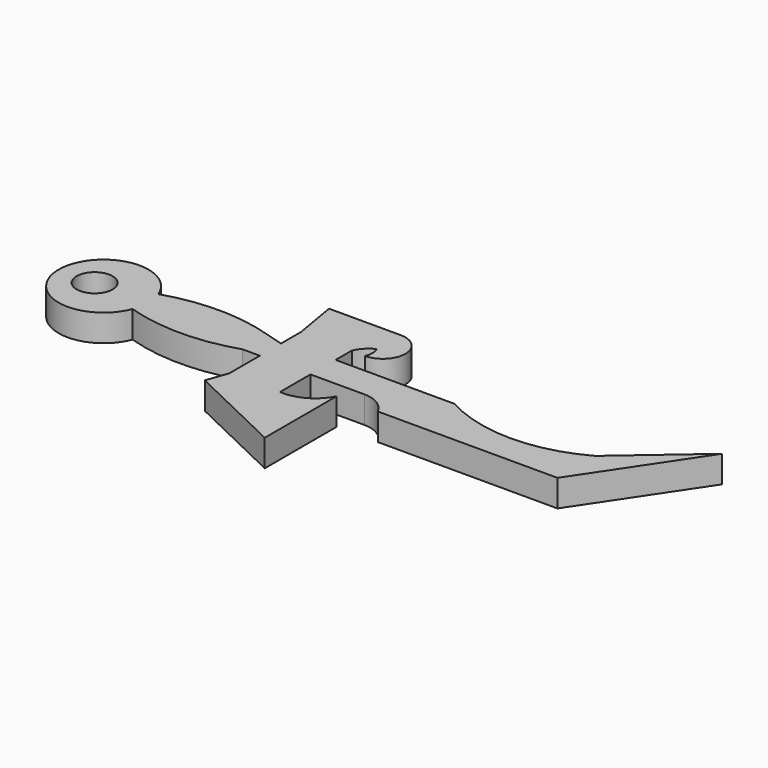
from build123d import *

# Parameters (mm, degrees)
F1_DEPTH = 3
F3_D     = 4


# Not quite as in the source:
# - a feature names something its author has since deleted; it is built from what else it names


with BuildPart() as f1:
    # F0 (on Top) → F1 (new body)
    with BuildSketch(Plane.XY):
        with BuildLine():
            Line((14.0881506171, 0), (14.0881506171, 3.5))
            ThreePointArc((14.0881506171, 3.5), (7.9876115371, 4.4807007673), (1.8788639221, 3.5525016304))
            ThreePointArc((1.8788639221, 3.5525016304), (2.1302987541, 2.666794093), (2.2150684857, 1.75))
            ThreePointArc((2.2150684857, 1.75), (2.1302987541, 0.833205907), (1.8788639221, -0.0525016304))
            ThreePointArc((1.8788639221, -0.0525016304), (7.9876115371, -0.9807007673), (14.0881506171, 0))
        make_face()
        with BuildLine():
            Line((21.6484292713, 3.5), (21.6484292713, 0))
            Line((21.6484292713, 0), (27.6484292713, 0))
            ThreePointArc((27.6484292713, 0), (29.3682210792, -0.4835632197), (30.5839958787, -1.7925356741))
            Line((30.5839958787, -1.7925356741), (50.5839958787, -1.7925356741))
            Line((50.5839958787, -1.7925356741), (58.9184745012, 10.6788903105))
            Line((58.9184745012, 10.6788903105), (50.5839958787, 3.5))
            ThreePointArc((50.5839958787, 3.5), (42.7439688076, 1.4762635236), (34.9039417364, 3.5))
            Line((34.9039417364, 3.5), (21.6484292713, 3.5))
        make_face()
        with BuildLine():
            Line((16.0120092332, 2.9430498835), (14.0881506171, 3.5))
            Line((14.0881506171, 3.5), (14.0881506171, 0))
            Line((14.0881506171, 0), (16.0120092332, 0))
            Line((16.0120092332, 0), (16.0120092332, -4.25))
            Line((16.0120092332, -4.25), (15.1717471866, -6.6045614651))
            Line((15.1717471866, -6.6045614651), (25.9923258961, -11.7925356741))
            Line((25.9923258961, -11.7925356741), (25.9923258961, -1.7925356741))
            ThreePointArc((25.9923258961, -1.7925356741), (24.192277602, -3.6786508222), (21.6484292713, -4.25))
            Line((21.6484292713, -4.25), (21.6484292713, 0))
            Line((21.6484292713, 0), (21.6484292713, 3.5))
            Line((21.6484292713, 3.5), (21.6484292713, 5.75))
            ThreePointArc((21.6484292713, 5.75), (22.2690927393, 6.6798640271), (23.1717471866, 7.3394739101))
            ThreePointArc((23.1717471866, 7.3394739101), (23.3522374925, 6.5091821103), (23.1717471866, 5.6788903105))
            ThreePointArc((23.1717471866, 5.6788903105), (25.6717471866, 8.1788903105), (23.1717471866, 10.6788903105))
            Line((23.1717471866, 10.6788903105), (15.1717471866, 10.6788903105))
            Line((15.1717471866, 10.6788903105), (16.0120092332, 5.75))
            Line((16.0120092332, 5.75), (16.0120092332, 2.9430498835))
        make_face()
        with BuildLine():
            ThreePointArc((1.7150684857, 3.5), (1.7969097631, 3.5264269002), (1.8788639221, 3.5525016304))
            ThreePointArc((1.8788639221, 3.5525016304), (-7.7849315143, 1.75), (1.8788639221, -0.0525016304))
            ThreePointArc((1.8788639221, -0.0525016304), (1.7969097631, -0.0264269002), (1.7150684857, 0))
            Line((1.7150684857, 0), (1.7150684857, 1.75))
            Line((1.7150684857, 1.75), (1.7150684857, 3.5))
        make_face()
        with BuildLine():
            ThreePointArc((2.2150684857, 1.75), (2.1302987541, 2.666794093), (1.8788639221, 3.5525016304))
            ThreePointArc((1.8788639221, 3.5525016304), (1.7969097631, 3.5264269002), (1.7150684857, 3.5))
            Line((1.7150684857, 3.5), (1.7150684857, 1.75))
            Line((1.7150684857, 1.75), (2.2150684857, 1.75))
        make_face()
        with BuildLine():
            ThreePointArc((1.8788639221, -0.0525016304), (2.1302987541, 0.833205907), (2.2150684857, 1.75))
            Line((2.2150684857, 1.75), (1.7150684857, 1.75))
            Line((1.7150684857, 1.75), (1.7150684857, 0))
            ThreePointArc((1.7150684857, 0), (1.7969097631, -0.0264269002), (1.8788639221, -0.0525016304))
        make_face()
    extrude(amount=F1_DEPTH)

    # F3 (through all)
    with Locations(Plane.XY.offset(3)):
        with Locations((-3.7849315143, 1.7499999964)):
            Hole(F3_D / 2)


solid = f1.part
